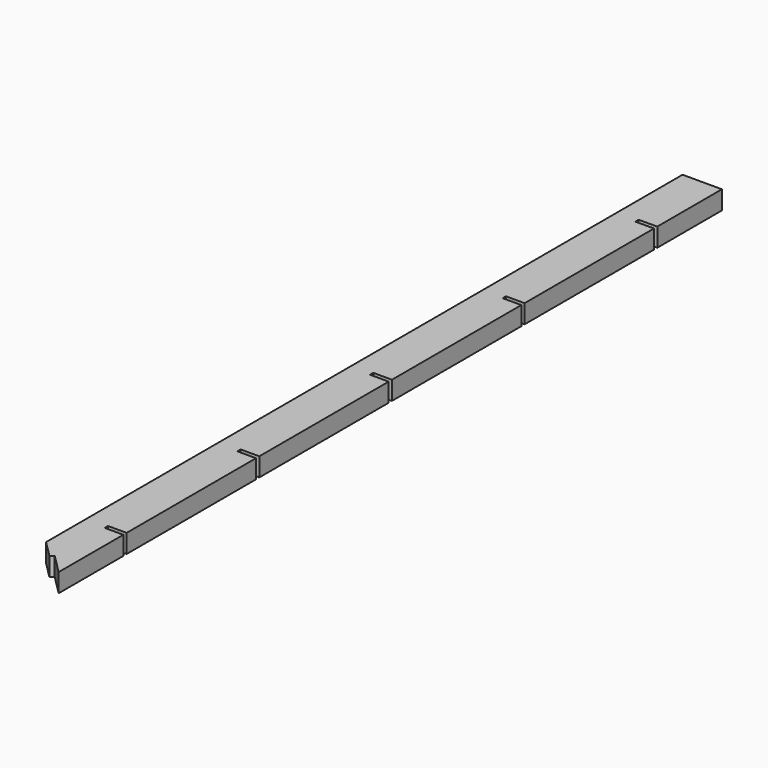
from build123d import *

# Parameters (mm, degrees)
F0_W            = 95
F0_H            = 45
F1_DEPTH        = 1250
F2_W            = 95
F2_H            = 250
F3_DEPTH        = 45
F5_DEPTH        = 5
F5_COPIES_COUNT = 3
F5_COPIES_PITCH = 400
F8_DEPTH        = 5
F11_DEPTH       = 5
F13_DEPTH       = 45


# Not quite as in the source:
# - a pattern or mirror of a feature is missing from the dataset's text; its kind, count and spacing are read off the source's solid


with BuildPart() as f1:
    # F0 (on Front) → F1 (new body, symmetric)
    with BuildSketch(Plane.XZ):
        Rectangle(F0_W, F0_H)
    extrude(amount=F1_DEPTH, both=True)

    # F2 (on face) → F3 (cut, through all)
    with BuildSketch(Plane.XY.offset(22.5)):
        with Locations((0, 1125)):
            Rectangle(F2_W, F2_H)
        Polygon((47.5, -1250), (47.5, -1000), (-47.5, -905), (-47.5, -1250), align=None)
    extrude(amount=-F3_DEPTH, mode=Mode.SUBTRACT)

    # F4 (on Front) → F5 (cut, symmetric)
    with BuildSketch(Plane.XZ):
        Polygon((47.5, 22.5), (2.5, 22.5), (2.5, 7.5), (32.5, 7.5), (32.5, -22.5), (47.5, -22.5), align=None)
    f5 = extrude(amount=F5_DEPTH, both=True, mode=Mode.SUBTRACT)

    # F5_copies: F5 ×3
    with Locations(*[(0, i * F5_COPIES_PITCH, 0) for i in range(1, F5_COPIES_COUNT)]):
        add(f5, mode=Mode.SUBTRACT)

    # F7 (on offset) → F8 (cut, symmetric)
    with BuildSketch(Plane.XZ.offset(800)):
        Polygon((2.5, 22.5), (2.5, 7.5), (32.5, 7.5), (32.5, -22.5), (47.5, -22.5), (47.5, 22.5), align=None)
    extrude(amount=F8_DEPTH, both=True, mode=Mode.SUBTRACT)

    # F10 (on offset) → F11 (cut, symmetric)
    with BuildSketch(Plane.XZ.offset(400)):
        Polygon((2.5, 22.5), (2.5, 7.5), (32.5, 7.5), (32.5, -22.5), (47.5, -22.5), (47.5, 22.5), align=None)
    extrude(amount=F11_DEPTH, both=True, mode=Mode.SUBTRACT)

    # F12 (on face) → F13 (join, through all)
    with BuildSketch(Plane.XY.offset(22.5)):
        Polygon((0, -952.5), (-47.5, -905), (-47.5, -919.1421356237), (-7.0710678119, -959.5710678119), align=None)
    extrude(amount=-F13_DEPTH)


solid = f1.part
